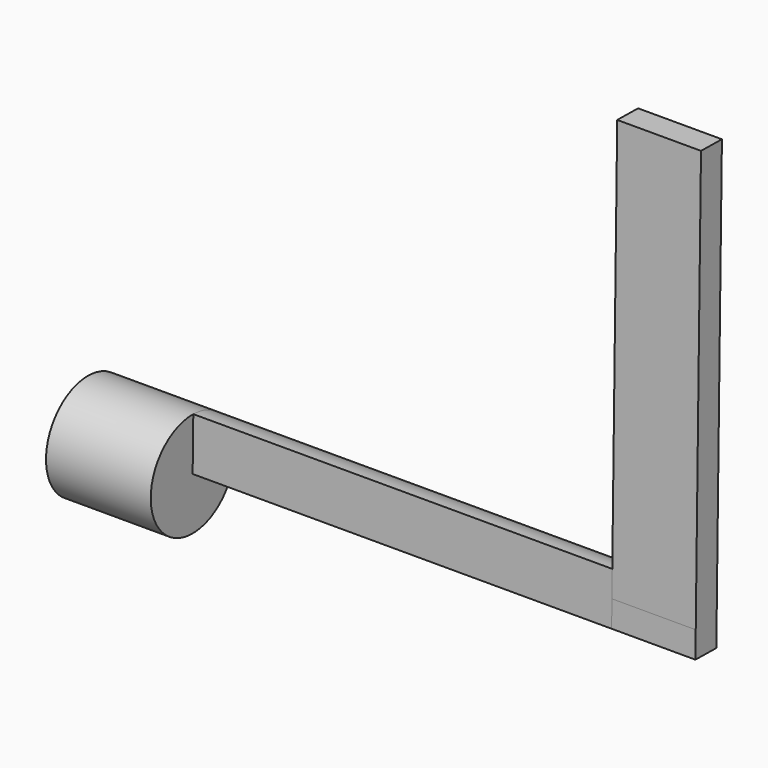
from build123d import *

# Parameters (mm, degrees)
F0_R     = 3.175
F1_DEPTH = 6.35
F5_DEPTH = 25.4
F7_DEPTH = 5.08
F8_DEPTH = 25.4


# Not quite as in the source:
# - the program builds the solid bodies; features that only make, move or delete a surface that nothing else refers to are left out


with BuildPart() as f1:
    # F0 (on Right) → F1 (new body)
    with BuildSketch(Plane.YZ):
        with Locations((-37.7712212503, 38.5835021734)):
            Circle(F0_R)
    extrude(amount=F1_DEPTH)

    # F4 (on face) → F5 (join)
    with BuildSketch(Plane.YZ.offset(6.35)):
        with BuildLine():
            ThreePointArc((-34.5962212503, 38.5835021734), (-35.5085896731, 40.8108601029), (-37.7213383186, 41.7581102899))
            Line((-37.7213383186, 41.7581102899), (-37.7712212503, 38.5835021734))
            Line((-37.7712212503, 38.5835021734), (-34.5966131338, 38.5336192417))
            ThreePointArc((-34.5966131338, 38.5336192417), (-34.5963192227, 38.5585599379), (-34.5962212503, 38.5835021734))
        make_face()
    extrude(amount=F5_DEPTH)

    # F6 (on face) → F7 (join)
    with BuildSketch(Plane.YZ.offset(31.75)):
        Polygon((-37.7712212503, 38.5835021734), (-36.1839171921, 38.5585607076), (-36.1610525797, 40.0136913835), (-36.1610525797, 40.1458973996), (-37.7462797844, 40.1708062317), align=None)
    extrude(amount=F7_DEPTH)

    # F8 (add): a face of the model
    f8_faces = [f1.faces().sort_by_distance(p)[0] for p in [
        (34.29, -36.953666182, 40.1583518156),
    ]]
    extrude(f8_faces, amount=F8_DEPTH)


solid = f1.part
